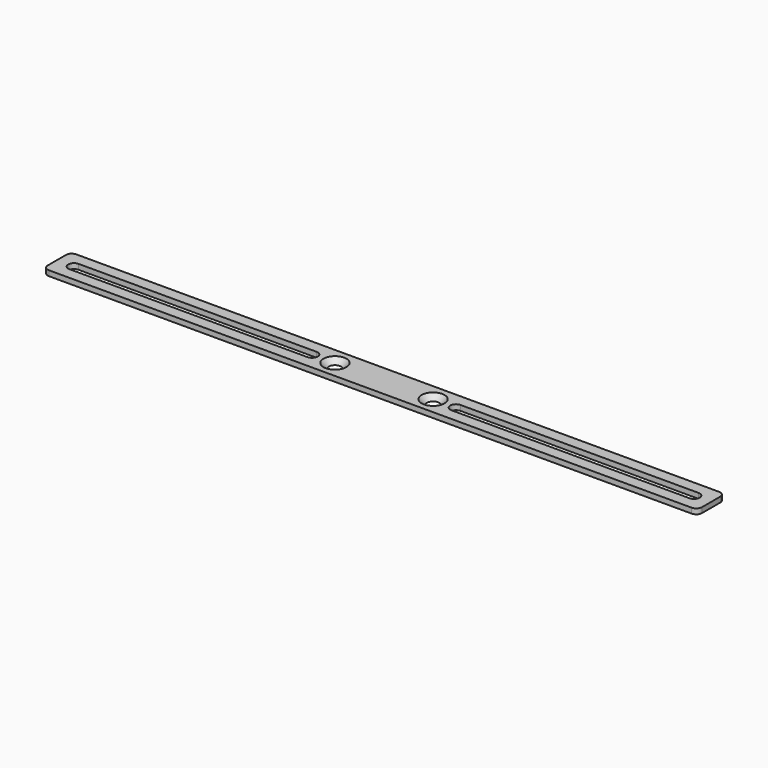
from build123d import *

# Parameters (mm, degrees)
F1_W     = 200
F1_H     = 10.5
F1_R     = 1.75
F2_DEPTH = 1.6
F3_R     = 1.75


# Not quite as in the source:
# - a fillet or chamfer that OpenCascade refuses, or shapes differently, is made with other operations: its cross-section is extruded or revolved along the edge and cut away or added
# - a feature names something its author has since deleted; it is built from what else it names


with BuildPart() as f2:
    # F1 (on Top) → F2 (new body)
    with BuildSketch(Plane.XY):
        with Locations((100, 5.25)):
            Rectangle(F1_W, F1_H)
        with BuildLine():
            ThreePointArc((78, 7), (79.75, 5.25), (78, 3.5))
            Line((78, 3.5), (5.25, 3.5))
            ThreePointArc((5.25, 3.5), (3.5, 5.25), (5.25, 7))
            Line((5.25, 7), (78, 7))
        make_face(mode=Mode.SUBTRACT)
        with Locations((85, 5.25)):
            Circle(F1_R, mode=Mode.SUBTRACT)
        with Locations((115, 5.25)):
            Circle(F1_R, mode=Mode.SUBTRACT)
        with BuildLine():
            Line((122, 7), (194.75, 7))
            ThreePointArc((194.75, 7), (196.5, 5.25), (194.75, 3.5))
            Line((194.75, 3.5), (122, 3.5))
            ThreePointArc((122, 3.5), (120.25, 5.25), (122, 7))
        make_face(mode=Mode.SUBTRACT)
    extrude(amount=F2_DEPTH)

    # F3
    f3_edges = [f2.edges().sort_by_distance(p)[0] for p in [
        (0, 10.5, 0.8),
        (0, 0, 0.8),
        (200, 0, 0.8),
        (200, 10.5, 0.8),
    ]]
    fillet(f3_edges, radius=F3_R)

    # F4: chamfer of 1.75 on 2 edges, made by hand

    # F4_s1 → F4_t2 (revolve, cut)
    with BuildSketch(Plane.XZ.offset(-5.25)):
        Polygon((88.5, 1.6), (86.75, -0.15), (86.75, 1.6), align=None)
    revolve(axis=Axis((85, 5.25, 1.6), (0, 0, 1)), mode=Mode.SUBTRACT)

    # F4_s3 → F4_t4 (revolve, cut)
    with BuildSketch(Plane.XZ.offset(-5.25)):
        Polygon((118.5, 1.6), (116.75, -0.15), (116.75, 1.6), align=None)
    revolve(axis=Axis((115, 5.25, 1.6), (0, 0, 1)), mode=Mode.SUBTRACT)


solid = f2.part
